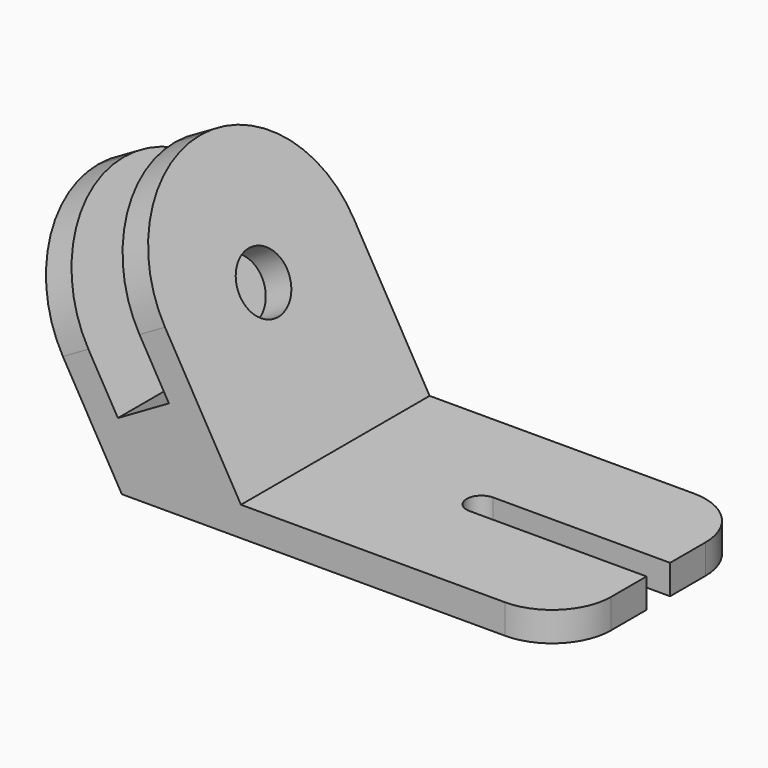
from build123d import *

# Parameters (mm, degrees)
F1_DEPTH = 80
F2_R     = 39.99999
F3_R     = 10
F4_DEPTH = 45
F6_DEPTH = 25
F7_R     = 20


# Not quite as in the source:
# - a fillet or chamfer is up to 0.001 mm smaller than in the source, because OpenCascade refuses the exact size


with BuildPart() as f1:
    # F0 (on Front) → F1 (new body)
    with BuildSketch(Plane.XZ):
        Polygon((-150, 0), (0, 0), (0, 10), (-109.5854811567, 10), (-155.3589838486, 89.2820323028), (-164.0192378865, 84.2820323028), (-134.0192378865, 32.3205080757), (-151.3397459622, 22.3205080757), (-181.3397459622, 74.2820323028), (-190, 69.2820323028), align=None)
    extrude(amount=F1_DEPTH)

    # F2 (radius 40 in the source; OpenCascade refuses exactly that, so slightly less here)
    f2_edges = [f1.edges().sort_by_distance(p)[0] for p in [
        (-159.689111, -80, 86.782032),
        (-159.689111, 0, 86.782032),
        (-185.669873, -80, 71.782032),
        (-185.669873, 0, 71.782032),
    ]]
    fillet(f2_edges, radius=F2_R)

    # F3 (on face) → F4 (cut)
    with BuildSketch(Plane(origin=(-77.8589838486, 0, -44.9519052838), x_dir=(0, 1, 0), z_dir=(0.8660254038, 0, 0.5))):
        with Locations((-40, 112.1529946162)):
            Circle(F3_R)
    extrude(amount=-F4_DEPTH, mode=Mode.SUBTRACT)

    # F5 (on face) → F6 (cut)
    with BuildSketch(Plane.XY.offset(10)):
        with BuildLine():
            Line((0, -40), (0, -35))
            Line((0, -35), (-60, -35))
            ThreePointArc((-60, -35), (-56.4644660941, -36.4644660941), (-55, -40))
            Line((-55, -40), (0, -40))
        make_face()
        with BuildLine():
            ThreePointArc((-55, -40), (-56.4644660941, -36.4644660941), (-60, -35))
            ThreePointArc((-60, -35), (-65, -40), (-60, -45))
            ThreePointArc((-60, -45), (-56.4644660941, -43.5355339059), (-55, -40))
        make_face()
        with BuildLine():
            Line((0, -45), (0, -40))
            Line((0, -40), (-55, -40))
            ThreePointArc((-55, -40), (-56.4644660941, -43.5355339059), (-60, -45))
            Line((-60, -45), (0, -45))
        make_face()
    extrude(amount=-F6_DEPTH, mode=Mode.SUBTRACT)

    # F7
    f7_edges = [f1.edges().sort_by_distance(p)[0] for p in [
        (0, -80, 5),
        (0, 0, 5),
    ]]
    fillet(f7_edges, radius=F7_R)


solid = f1.part
